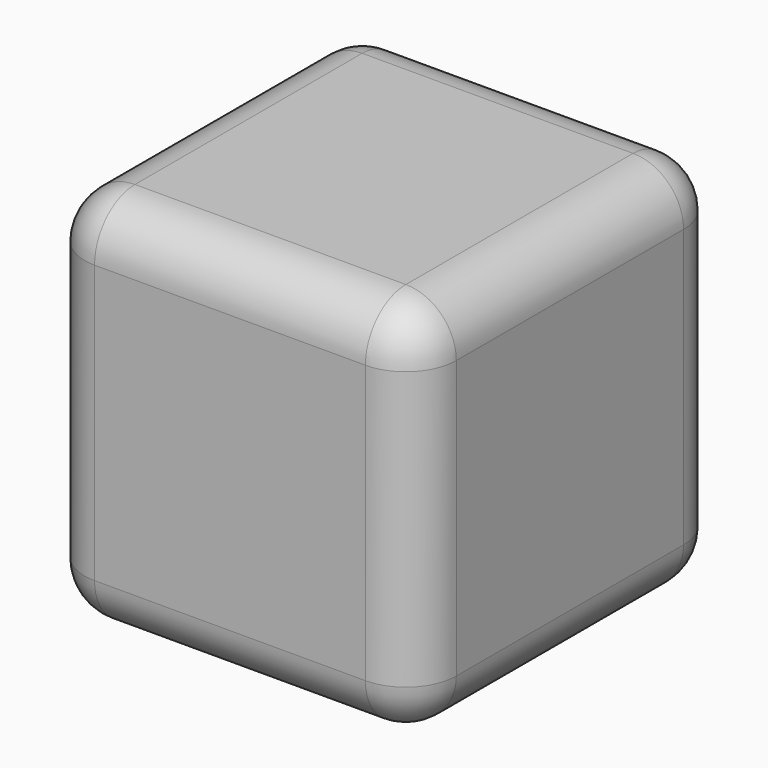
from build123d import *

# Parameters (mm, degrees)
F0_W     = 37.4110154808
F0_H     = 38.7368313968
F1_DEPTH = 38.1
F2_R     = 5.08
F3_R     = 5.08
F4_R     = 5.08
F5_R     = 5.08
F6_R     = 5.08
F7_R     = 5.08


# Not quite as in the source:
# - the program builds the solid bodies; features that only make, move or delete a surface that nothing else refers to are left out


with BuildPart() as f1:
    # F0 (on Top) → F1 (new body)
    with BuildSketch(Plane.XY):
        Rectangle(F0_W, F0_H)
    extrude(amount=F1_DEPTH)

    # F2
    f2_edges = [f1.edges().sort_by_distance(p)[0] for p in [
        (18.705508, -19.368416, 19.05),
    ]]
    fillet(f2_edges, radius=F2_R)

    # F3
    f3_edges = [f1.edges().sort_by_distance(p)[0] for p in [
        (-18.705508, -19.368416, 19.05),
    ]]
    fillet(f3_edges, radius=F3_R)

    # F4
    f4_edges = [f1.edges().sort_by_distance(p)[0] for p in [
        (-18.705508, 19.368416, 19.05),
    ]]
    fillet(f4_edges, radius=F4_R)

    # F5
    f5_edges = [f1.edges().sort_by_distance(p)[0] for p in [
        (18.705508, 19.368416, 19.05),
    ]]
    fillet(f5_edges, radius=F5_R)

    # F6
    f6_edges = [f1.edges().sort_by_distance(p)[0] for p in [
        (0, 19.368416, 38.1),
    ]]
    fillet(f6_edges, radius=F6_R)

    # F7
    f7_edges = [f1.edges().sort_by_distance(p)[0] for p in [
        (0, -19.368416, 0),
    ]]
    fillet(f7_edges, radius=F7_R)


solid = f1.part
